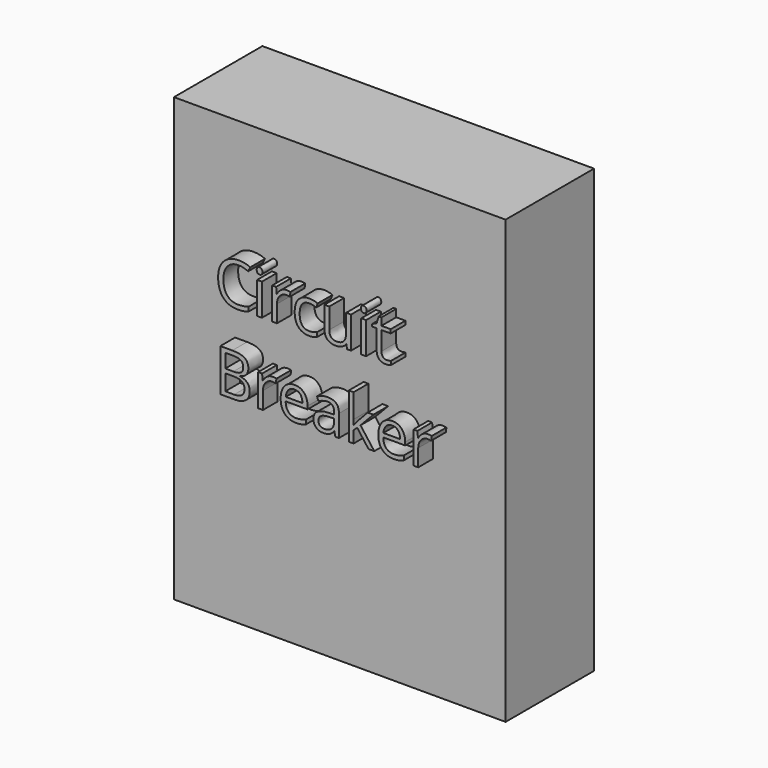
from build123d import *

# Parameters (mm, degrees)
F0_W         = 457.2
F0_H         = 609.6
F1_DEPTH     = 152.4
F2_TEXT_SIZE = 81.9733579863
F3_DEPTH     = 25.4


# Not quite as in the source:
# - Text() gives the source's letters only with a copy of the font that has no kerning and outlines rounded to 1/6400 em; it was checked with that copy


with BuildPart() as f1:
    # F0 (on Front) → F1 (new body)
    with BuildSketch(Plane.XZ):
        Rectangle(F0_W, F0_H)
    extrude(amount=F1_DEPTH)

    # F2 (on face) → F3 (join)
    with BuildSketch(Plane.XZ.offset(152.4)):
        with Locations((-152.4, 93.3791822499)):
            Text('Circuit', F2_TEXT_SIZE, font='Open Sans', text_align=(TextAlign.LEFT, TextAlign.BOTTOM))
        with Locations((-152.4, -18.1045846115)):
            Text('Breaker', F2_TEXT_SIZE, font='Open Sans', text_align=(TextAlign.LEFT, TextAlign.BOTTOM))
    extrude(amount=F3_DEPTH)


solid = f1.part
